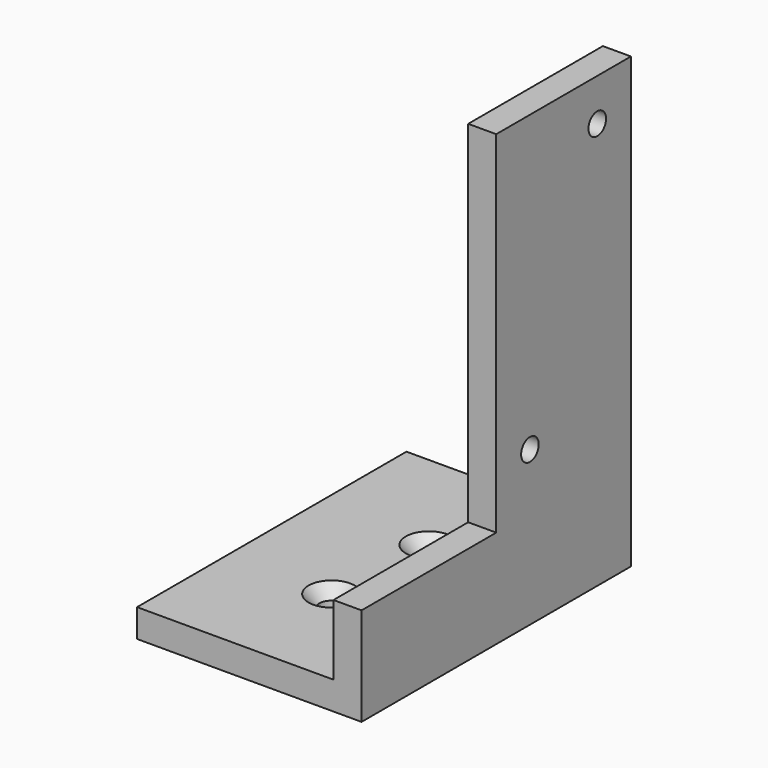
from build123d import *

# Parameters (mm, degrees)
F1_DEPTH       = 76.2
F3_D           = 4.9784
F3_CSINK_D     = 9.1186
F3_CSINK_ANGLE = 82
F5_D           = 5.6134
F5_CSINK_D     = 10.4394
F5_CSINK_ANGLE = 82
F6_W           = 38.1
F6_H           = 79.375
F7_DEPTH       = 6.351


# Not quite as in the source:
# - a feature names something its author has since deleted; it is built from what else it names


with BuildPart() as f1:
    # F0 (on Front) → F1 (new body)
    with BuildSketch(Plane.XZ):
        Polygon((-50.8, 0), (0, 0), (0, 101.6), (-6.35, 101.6), (-6.35, 6.35), (-50.8, 6.35), align=None)
    extrude(amount=F1_DEPTH)

    # F3 (through all)
    with Locations(Plane(origin=(-6.35, 0, 0), x_dir=(0, -1, 0), z_dir=(-1, 0, 0))):
        with Locations((9.525, 92.075), (28.575, 34.925)):
            CounterSinkHole(F3_D / 2, F3_CSINK_D / 2, counter_sink_angle=F3_CSINK_ANGLE)

    # F5 (through all)
    with Locations(Plane.XY.offset(6.35)):
        with Locations((-25.4, -25.4), (-27.0796256672, -50.8)):
            CounterSinkHole(F5_D / 2, F5_CSINK_D / 2, counter_sink_angle=F5_CSINK_ANGLE)

    # F6 (on face) → F7 (cut, through all)
    with BuildSketch(Plane(origin=(-6.35, 0, 0), x_dir=(0, -1, 0), z_dir=(-1, 0, 0))):
        with Locations((57.15, 61.9125)):
            Rectangle(F6_W, F6_H)
    extrude(amount=-F7_DEPTH, mode=Mode.SUBTRACT)


solid = f1.part
